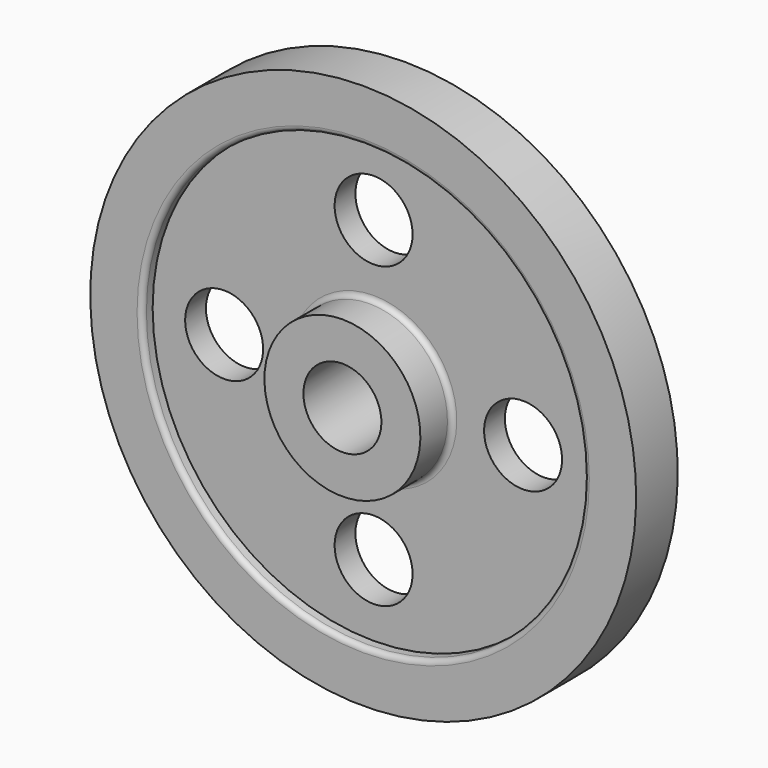
from build123d import *

# Parameters (mm, degrees)
F2_R     = 19.05
F3_DEPTH = 25.4
F4_R     = 2.54


# Not quite as in the source:
# - a feature of the source that left no trace in its solid (it failed there, or was rolled back) is left out


with BuildPart() as f1:
    # F0 (on Right) → F1 (revolve)
    with BuildSketch(Plane.YZ):
        Polygon((-25.4, 19.05), (0, 19.05), (25.4, 19.05), (25.4, 38.1), (6.35, 38.1), (6.35, 107.95), (12.7, 107.95), (12.7, 133.35), (6.35, 133.35), (0, 133.35), (-12.7, 133.35), (-12.7, 107.95), (-6.35, 107.95), (-6.35, 38.1), (-25.4, 38.1), align=None)
    revolve(axis=Axis((0, 38.1000004709, 0), (0, 1, 0)))

    # F2 (on face) → F3 (cut)
    with BuildSketch(Plane(origin=(0, 6.35, 0), x_dir=(-1, 0, 0), z_dir=(0, 1, 0))):
        with BuildLine():
            ThreePointArc((19.05, 73.025), (-13.4703841816, 86.4953841816), (0, 53.975))
            ThreePointArc((0, 53.975), (13.4703841816, 59.5546158184), (19.05, 73.025))
        make_face()
        with Locations((73.025, 0)):
            Circle(F2_R)
        with Locations((0, -73.025)):
            Circle(F2_R)
        with Locations((-73.025, 0)):
            Circle(F2_R)
    extrude(amount=-F3_DEPTH, mode=Mode.SUBTRACT)

    # F4
    f4_edges = [f1.edges().sort_by_distance(p)[0] for p in [
        (0, 25.4, -19.05),
        (0, 25.4, -38.1),
        (0, 12.7, -107.95),
        (0, -6.35, -38.1),
        (0, -12.7, -107.95),
    ]]
    fillet(f4_edges, radius=F4_R)


solid = f1.part
